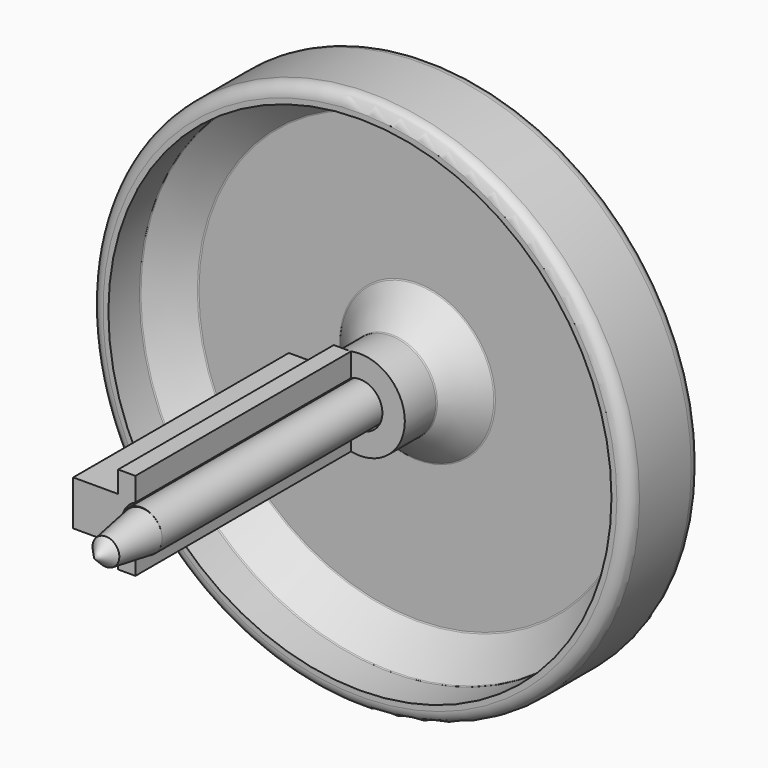
from build123d import *

# Parameters (mm, degrees)
F0_R      = 19.05
F1_DEPTH  = 6.35
F2_R      = 17.78
F2_R_2    = 3.175
F3_DEPTH  = 5.08
F4_R      = 1.5875
F5_DEPTH  = 6.35
F6_R      = 3.175
F7_DEPTH  = 0.254
F8_R      = 1.4605
F9_DEPTH  = 25.4
F12_R     = 2.921
F13_DEPTH = 0.4826
F14_R     = 0.25399
F14_2_R   = 0.25399
F15_R     = 0.889
F16_SIZE  = 2.286
F17_R     = 0.127
F19_DEPTH = 19.05


# Not quite as in the source:
# - a fillet or chamfer is up to 0.001 mm smaller than in the source, because OpenCascade refuses the exact size


with BuildPart() as f1:
    # F0 (on Front) → F1 (new body)
    with BuildSketch(Plane.XZ):
        with Locations((0.6285069608, 0)):
            Circle(F0_R)
    extrude(amount=F1_DEPTH)

    # F2 (on face) → F3 (cut)
    with BuildSketch(Plane.XZ.offset(6.35)):
        with Locations((0.6285069608, 0)):
            Circle(F2_R)
        with Locations((0.6285069608, 0)):
            Circle(F2_R_2, mode=Mode.SUBTRACT)
    extrude(amount=-F3_DEPTH, mode=Mode.SUBTRACT)

    # F4 (on face) → F5 (cut, through all)
    with BuildSketch(Plane.XZ.offset(6.35)):
        with Locations((0.6285069608, 0)):
            Circle(F4_R)
    extrude(amount=-F5_DEPTH, mode=Mode.SUBTRACT)

    # F6 (on face) → F7 (cut)
    with BuildSketch(Plane(origin=(0, 0, 0), x_dir=(-1, 0, 0), z_dir=(0, 1, 0))):
        with Locations((-0.6285069608, 0)):
            Circle(F6_R)
    extrude(amount=-F7_DEPTH, mode=Mode.SUBTRACT)

    # F14 (radius 0.254 in the source; OpenCascade refuses exactly that, so slightly less here)
    f14_edges = [f1.edges().sort_by_distance(p)[0] for p in [
        (3.803507, 0, 0),
    ]]
    fillet(f14_edges, radius=F14_R)

    # F15
    f15_edges = [f1.edges().sort_by_distance(p)[0] for p in [
        (-18.421493, 0, 0),
        (-18.421493, -6.35, 0),
    ]]
    fillet(f15_edges, radius=F15_R)

    # F16
    f16_edges = [f1.edges().sort_by_distance(p)[0] for p in [
        (-17.151493, -1.27, 0),
        (-2.546493, -1.27, 0),
    ]]
    chamfer(f16_edges, length=F16_SIZE)

    # F17
    f17_edges = [f1.edges().sort_by_distance(p)[0] for p in [
        (-14.865493, -1.27, 0),
        (-4.832493, -1.27, 0),
        (-2.546493, -3.556, 0),
        (-17.151493, -3.556, 0),
    ]]
    fillet(f17_edges, radius=F17_R)


with BuildPart() as f9:
    # F8 (on face) → F9 (new body)
    with BuildSketch(Plane(origin=(0, -0.254, 0), x_dir=(-1, 0, 0), z_dir=(0, 1, 0))):
        with Locations((-0.6285069608, 0)):
            Circle(F8_R)
    extrude(amount=-F9_DEPTH)

    # F10 (on Top) → F11 (revolve)
    with BuildSketch(Plane.XY):
        Polygon((2.0889979787, -25.654), (0.6578754546, -25.654), (0.6578754546, -29.8726570247), (1.605724523, -28.8281862079), align=None)
    revolve(axis=Axis((0.6578754546, -27.7633285124, 0), (0, -1, 0)))

    # F12 (on face) → F13 (join)
    with BuildSketch(Plane(origin=(0, -0.254, 0), x_dir=(-1, 0, 0), z_dir=(0, 1, 0))):
        with Locations((-0.6285069608, 0)):
            Circle(F12_R)
    extrude(amount=F13_DEPTH)

    # F14#2 (radius 0.254 in the source; OpenCascade refuses exactly that, so slightly less here)
    f14_2_edges = [f9.edges().sort_by_distance(p)[0] for p in [
        (3.549507, 0.2286, 0),
    ]]
    fillet(f14_2_edges, radius=F14_2_R)


with BuildPart() as f19:
    # F18 (on face) → F19 (new body)
    with BuildSketch(Plane.XZ.offset(6.35)):
        with BuildLine():
            Line((0, 1.4577843634), (0, 3.1121703039))
            Line((0, 3.1121703039), (-1.2189875124, 3.1121703039))
            Line((-1.2189875124, 3.1121703039), (-1.2189875124, 1.5875))
            Line((-1.2189875124, 1.5875), (-4.3939875124, 1.5875))
            Line((-4.3939875124, 1.5875), (-4.3939875124, -1.5875))
            Line((-4.3939875124, -1.5875), (-1.2189875124, -1.5875))
            Line((-1.2189875124, -1.5875), (-1.2189875124, -3.1121703039))
            Line((-1.2189875124, -3.1121703039), (0, -3.1121703039))
            Line((0, -3.1121703039), (0, -1.4577843634))
            ThreePointArc((0, -1.4577843634), (-0.9589930392, 0), (0, 1.4577843634))
        make_face()
    extrude(amount=F19_DEPTH)


solid = Compound([f1.part, f9.part, f19.part])
